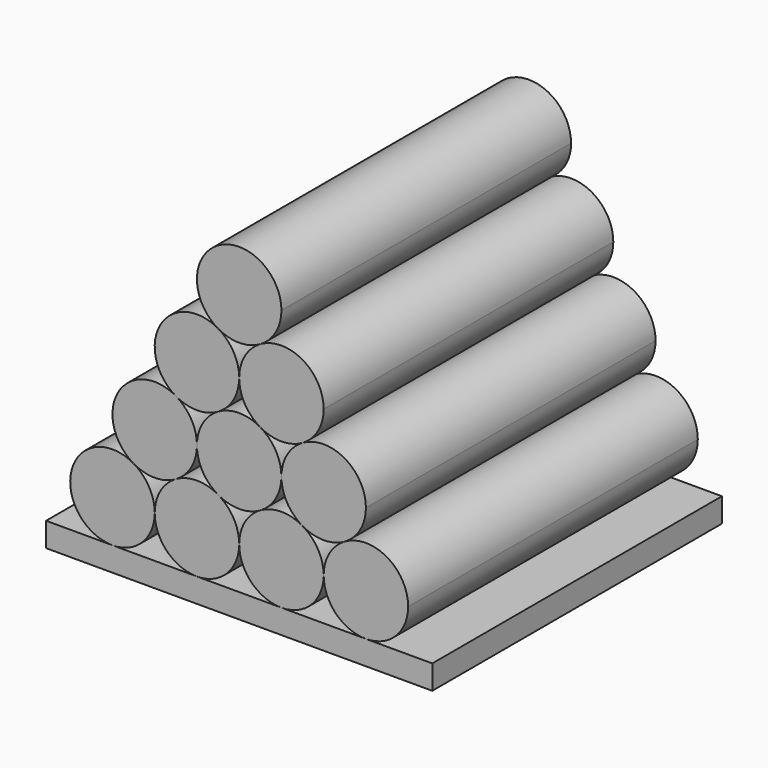
from build123d import *

# Parameters (mm, degrees)
F1_DEPTH = 76.2


# Not quite as in the source:
# - a feature names something its author has since deleted; it is built from what else it names


with BuildPart() as f1:
    # F0 (on Front) → F1 (new body)
    with BuildSketch(Plane.XZ):
        with BuildLine():
            ThreePointArc((-22.2250001435, -7.6989659225), (-18.9710342018, -4.4450000718), (-17.78, 0))
            ThreePointArc((-17.78, 0), (-18.9710341832, 4.4450000396), (-22.2250000791, 7.6989658853))
            ThreePointArc((-22.2250000791, 7.6989658853), (-34.3689658613, 4.4449999625), (-31.1150000042, -7.6989658372))
            ThreePointArc((-31.1150000042, -7.6989658372), (-26.6700000853, -8.89), (-22.2250001435, -7.6989659225))
        make_face()
    extrude(amount=F1_DEPTH)


with BuildPart() as f1b:
    # F0 (on Front) → F1, piece 2 (new body)
    with BuildSketch(Plane.XZ):
        with BuildLine():
            ThreePointArc((-13.3350000511, 7.6989658101), (-16.5889658544, 4.4449999744), (-17.78, 0))
            ThreePointArc((-17.78, 0), (-16.5889658625, -4.4449999603), (-13.3350000793, -7.6989657939))
            ThreePointArc((-13.3350000793, -7.6989657939), (-8.8900000289, -8.89), (-4.4449999708, -7.6989658228))
            ThreePointArc((-4.4449999708, -7.6989658228), (-1.1910341519, -4.4449999854), (0, 0))
            ThreePointArc((0, 0), (-1.1910341518, 4.4449999853), (-4.4449999705, 7.6989658226))
            ThreePointArc((-4.4449999705, 7.6989658226), (-8.8900000125, 8.89), (-13.3350000511, 7.6989658101))
        make_face()
    extrude(amount=F1_DEPTH)


with BuildPart() as f1c:
    # F0 (on Front) → F1, piece 3 (new body)
    with BuildSketch(Plane.XZ):
        with BuildLine():
            ThreePointArc((-13.3350001127, 23.096897584), (-25.4789658493, 19.8429316625), (-22.2250000791, 7.6989658853))
            ThreePointArc((-22.2250000791, 7.6989658853), (-17.7800000752, 6.5079316793), (-13.3350000511, 7.6989658101))
            ThreePointArc((-13.3350000511, 7.6989658101), (-10.0810341751, 10.9529316537), (-8.89, 15.3979316793))
            ThreePointArc((-8.89, 15.3979316793), (-10.0810341929, 19.8429317356), (-13.3350001127, 23.096897584))
        make_face()
    extrude(amount=F1_DEPTH)


with BuildPart() as f1d:
    # F0 (on Front) → F1, piece 4 (new body)
    with BuildSketch(Plane.XZ):
        with BuildLine():
            ThreePointArc((-13.3350000793, -7.6989657939), (-17.7800001286, -6.5079316793), (-22.2250001435, -7.6989659225))
            ThreePointArc((-22.2250001435, -7.6989659225), (-25.4789658811, -10.952931751), (-26.67, -15.3979316793))
            ThreePointArc((-26.67, -15.3979316793), (-24.0661792847, -21.684110964), (-17.78, -24.2879316793))
            ThreePointArc((-17.78, -24.2879316793), (-11.4938207153, -21.684110964), (-8.89, -15.3979316793))
            ThreePointArc((-8.89, -15.3979316793), (-10.0810341832, -10.9529316396), (-13.3350000793, -7.6989657939))
        make_face()
    extrude(amount=F1_DEPTH)


with BuildPart() as f1e:
    # F0 (on Front) → F1, piece 5 (new body)
    with BuildSketch(Plane.XZ):
        with BuildLine():
            ThreePointArc((-26.67, -15.3979316793), (-27.8610341616, -10.9529316772), (-31.1150000042, -7.6989658372))
            ThreePointArc((-31.1150000042, -7.6989658372), (-44.1470805963, -13.0970303707), (-35.56, -24.2879316793))
            ThreePointArc((-35.56, -24.2879316793), (-29.2738207153, -21.684110964), (-26.67, -15.3979316793))
        make_face()
    extrude(amount=F1_DEPTH)


with BuildPart() as f1f:
    # F0 (on Front) → F1, piece 6 (new body)
    with BuildSketch(Plane.XZ):
        with BuildLine():
            ThreePointArc((0, 30.7958633586), (-13.3349999436, 38.4948292308), (-13.3350001127, 23.096897584))
            ThreePointArc((-13.3350001127, 23.096897584), (-8.8900000658, 21.9058633586), (-4.4450000013, 23.0968975182))
            ThreePointArc((-4.4450000013, 23.0968975182), (-1.1910341607, 26.3508633579), (0, 30.7958633586))
        make_face()
    extrude(amount=F1_DEPTH)


with BuildPart() as f1g:
    # F0 (on Front) → F1, piece 7 (new body)
    with BuildSketch(Plane.XZ):
        with BuildLine():
            ThreePointArc((-8.89, 15.3979316793), (-7.6989658311, 10.9529316645), (-4.4449999705, 7.6989658226))
            ThreePointArc((-4.4449999705, 7.6989658226), (6.75e-08, 6.5079316793), (4.4450000875, 7.6989658901))
            ThreePointArc((4.4450000875, 7.6989658901), (7.6989658649, 10.952931723), (8.89, 15.3979316793))
            ThreePointArc((8.89, 15.3979316793), (4.4449999993, 23.0968975193), (-4.4450000013, 23.0968975182))
            ThreePointArc((-4.4450000013, 23.0968975182), (-7.69896584, 19.8429316786), (-8.89, 15.3979316793))
        make_face()
    extrude(amount=F1_DEPTH)


with BuildPart() as f1h:
    # F0 (on Front) → F1, piece 8 (new body)
    with BuildSketch(Plane.XZ):
        with BuildLine():
            ThreePointArc((4.4450000013, -7.6989658404), (1.76e-08, -6.5079316793), (-4.4449999708, -7.6989658228))
            ThreePointArc((-4.4449999708, -7.6989658228), (-7.6989658312, -10.9529316647), (-8.89, -15.3979316793))
            ThreePointArc((-8.89, -15.3979316793), (-6.2861793033, -21.6841109454), (-5.26e-08, -24.2879316793))
            ThreePointArc((-5.26e-08, -24.2879316793), (6.2861792662, -21.6841109826), (8.89, -15.3979316793))
            ThreePointArc((8.89, -15.3979316793), (7.69896584, -10.9529316799), (4.4450000013, -7.6989658404))
        make_face()
    extrude(amount=F1_DEPTH)


with BuildPart() as f1i:
    # F0 (on Front) → F1, piece 9 (new body)
    with BuildSketch(Plane.XZ):
        Polygon((-17.78, -24.2879316793), (-35.56, -24.2879316793), (-49.53, -24.2879316793), (-49.53, -29.3679316793), (31.75, -29.3679316793), (31.75, -24.2879316793), (17.7799999808, -24.2879316793), (-5.26e-08, -24.2879316793), align=None)
    extrude(amount=F1_DEPTH)


with BuildPart() as f1j:
    # F0 (on Front) → F1, piece 10 (new body)
    with BuildSketch(Plane.XZ):
        with BuildLine():
            ThreePointArc((4.4450000875, 7.6989658901), (1.1910341856, 4.4450000437), (0, 0))
            ThreePointArc((0, 0), (1.1910341607, -4.4450000007), (4.4450000013, -7.6989658404))
            ThreePointArc((4.4450000013, -7.6989658404), (8.8899999644, -8.89), (13.3349999371, -7.698965876))
            ThreePointArc((13.3349999371, -7.698965876), (16.5889658215, -4.4450000314), (17.78, 0))
            ThreePointArc((17.78, 0), (13.3350000437, 7.6989658144), (4.4450000875, 7.6989658901))
        make_face()
    extrude(amount=F1_DEPTH)


with BuildPart() as f1k:
    # F0 (on Front) → F1, piece 11 (new body)
    with BuildSketch(Plane.XZ):
        with BuildLine():
            ThreePointArc((26.67, -15.3979316793), (22.2249999686, -7.6989658215), (13.3349999371, -7.698965876))
            ThreePointArc((13.3349999371, -7.698965876), (10.0810341422, -10.9529317107), (8.89, -15.3979316793))
            ThreePointArc((8.89, -15.3979316793), (11.4938207085, -21.6841109572), (17.7799999808, -24.2879316793))
            ThreePointArc((17.7799999808, -24.2879316793), (24.066179278, -21.6841109708), (26.67, -15.3979316793))
        make_face()
    extrude(amount=F1_DEPTH)


solid = Compound([f1.part, f1b.part, f1c.part, f1d.part, f1e.part, f1f.part, f1g.part, f1h.part, f1i.part, f1j.part, f1k.part])
